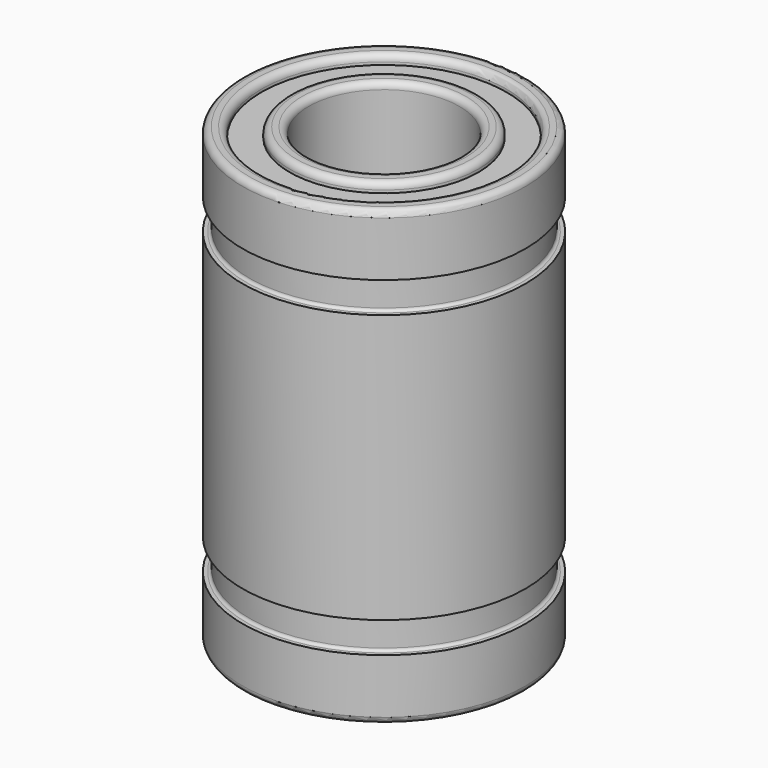
from build123d import *

# Parameters (mm, degrees)
F1_R     = 7.5
F1_R_2   = 6.5
F2_DEPTH = 24
F3_R     = 5
F3_R_2   = 4
F4_DEPTH = 24
F5_R     = 0.35
F5_2_R   = 0.35
F7_START = 0.5
F6_R     = 6.5
F6_R_2   = 5
F7_DEPTH = 23
F8_W     = 4.3079123679
F8_H     = 1.6359793772
F10_R    = 0.15


with BuildPart() as f2:
    # F1 (on Top) → F2 (new body, through all)
    with BuildSketch(Plane.XY):
        Circle(F1_R)
        Circle(F1_R_2, mode=Mode.SUBTRACT)
    extrude(amount=F2_DEPTH)

    # F5
    f5_edges = [f2.edges().sort_by_distance(p)[0] for p in [
        (-7.5, 0, 24),
        (-7.5, 0, 0),
        (-6.5, 0, 24),
        (-6.5, 0, 0),
    ]]
    fillet(f5_edges, radius=F5_R)



with BuildPart() as f4:
    # F3 (on Top) → F4 (new body, through all)
    with BuildSketch(Plane.XY):
        Circle(F3_R)
        Circle(F3_R_2, mode=Mode.SUBTRACT)
    extrude(amount=F4_DEPTH)

    # F5#2
    f5_2_edges = [f4.edges().sort_by_distance(p)[0] for p in [
        (-5, 0, 0),
        (-4, 0, 0),
        (-5, 0, 24),
        (-4, 0, 24),
    ]]
    fillet(f5_2_edges, radius=F5_2_R)


with BuildPart() as f2_1:
    add(f2.part)

    add(f4.part)  # F7 merges F4
    # F6 (on Top) → F7 (join)
    with BuildSketch(Plane.XY.offset(F7_START)):
        Circle(F6_R)
        Circle(F6_R_2, mode=Mode.SUBTRACT)
    extrude(amount=F7_DEPTH)

    # F8 (on Front) → F9 (revolve, cut)
    with BuildSketch(Plane.XZ):
        with Locations((9.303956184, 19.9320103114)):
            Rectangle(F8_W, F8_H)
        with Locations((9.303956184, 4.0679896886)):
            Rectangle(F8_W, F8_H)
    revolve(axis=Axis((0, 0, 0), (0, 0, -1)), mode=Mode.SUBTRACT)

    # F10
    f10_edges = [f2_1.edges().sort_by_distance(p)[0] for p in [
        (-7.15, 0, 20.75),
        (-7.15, 0, 19.114021),
        (-7.15, 0, 3.25),
        (-7.15, 0, 4.885979),
    ]]
    fillet(f10_edges, radius=F10_R)


solid = f2_1.part
